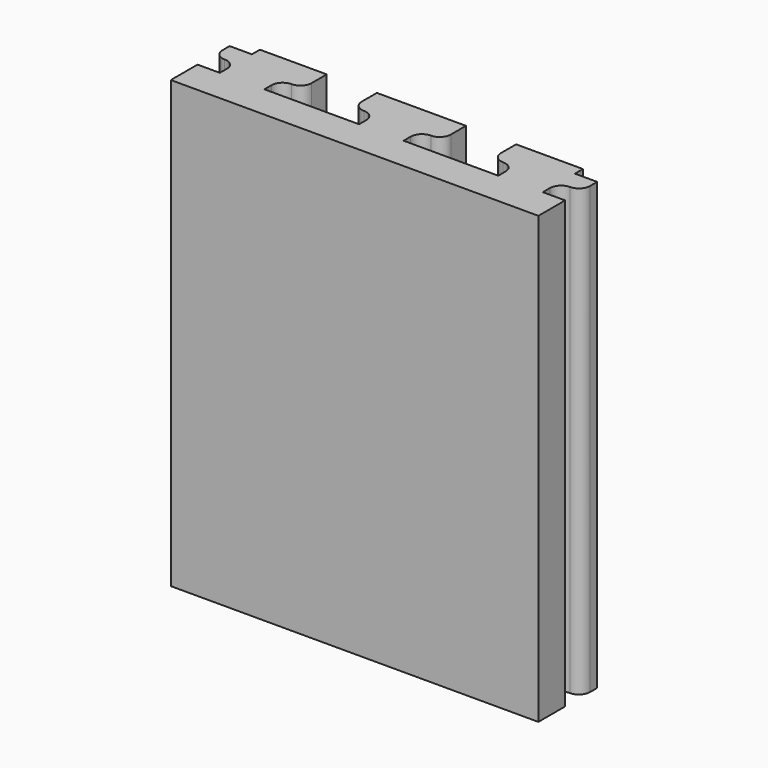
from build123d import *

# Parameters (mm, degrees)
F0_W     = 4
F0_H     = 1.8
F0_W_2   = 2
F1_DEPTH = 20
F2_R     = 0.99999


# Not quite as in the source:
# - a fillet or chamfer is up to 0.001 mm smaller than in the source, because OpenCascade refuses the exact size


with BuildPart() as f1:
    # F0 (on Top) → F1 (new body, symmetric)
    with BuildSketch(Plane.XY):
        Polygon((-2, 1.1054119891), (-2, 0.2054119891), (2, 0.2054119891), (4, 0.2054119891), (4, 1.1054119891), align=None)
        with Locations((0, -0.6945880109)):
            Rectangle(F0_W, F0_H)
        with Locations((-3, -0.6945880109)):
            Rectangle(F0_W_2, F0_H)
        with Locations((3, -0.6945880109)):
            Rectangle(F0_W_2, F0_H)
        with Locations((0, -2.4945880109)):
            Rectangle(F0_W, F0_H)
        Polygon((2, -3.3945880109), (-2, -3.3945880109), (-4, -3.3945880109), (-4, -6.3945880109), (29, -6.3945880109), (29, -3.3945880109), (27, -3.3945880109), (23, -3.3945880109), (14.5, -3.3945880109), (10.5, -3.3945880109), align=None)
        with Locations((12.5, -2.4945880109)):
            Rectangle(F0_W, F0_H)
        with Locations((12.5, -0.6945880109)):
            Rectangle(F0_W, F0_H)
        with Locations((9.5, -0.6945880109)):
            Rectangle(F0_W_2, F0_H)
        with Locations((15.5, -0.6945880109)):
            Rectangle(F0_W_2, F0_H)
        with Locations((25, -2.4945880109)):
            Rectangle(F0_W, F0_H)
        Polygon((8.5, 0.2054119891), (10.5, 0.2054119891), (14.5, 0.2054119891), (16.5, 0.2054119891), (16.5, 1.1054119891), (8.5, 1.1054119891), align=None)
        with Locations((25, -0.6945880109)):
            Rectangle(F0_W, F0_H)
        with Locations((22, -0.6945880109)):
            Rectangle(F0_W_2, F0_H)
        with Locations((28, -0.6945880109)):
            Rectangle(F0_W_2, F0_H)
        Polygon((21, 0.2054119891), (23, 0.2054119891), (27, 0.2054119891), (27, 1.1054119891), (21, 1.1054119891), align=None)
    extrude(amount=F1_DEPTH, both=True)

    # F2 (radius 1 in the source; OpenCascade refuses exactly that, so slightly less here)
    f2_edges = [f1.edges().sort_by_distance(p)[0] for p in [
        (-2, -1.594588, 0),
        (2, -1.594588, 0),
        (10.5, -1.594588, 0),
        (14.5, -1.594588, 0),
        (23, -1.594588, 0),
        (27, -1.594588, 0),
        (8.5, -1.594588, 0),
        (-4, -1.594588, 0),
        (21, -1.594588, 0),
        (16.5, -1.594588, 0),
        (29, -1.594588, 0),
        (4, -1.594588, 0),
    ]]
    fillet(f2_edges, radius=F2_R)


solid = f1.part
